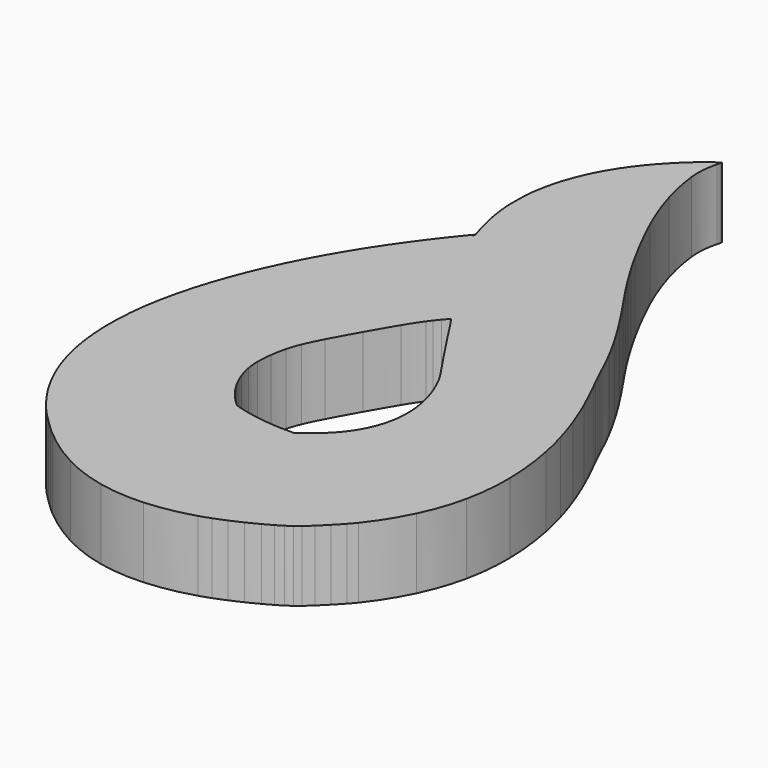
from build123d import *

# Parameters (mm, degrees)
F1_DEPTH = 7


# Not quite as in the source:
# - ends of sketch curves that miss each other by under 0.0002 mm in the source are joined


with BuildPart() as f1:
    # F0 (on Top) → F1 (new body)
    with BuildSketch(Plane.XY):
        with BuildLine():
            ThreePointArc((-0.430785183, 36.1569095573), (-0.5448735218, 36.07329488), (-0.6583357739, 35.9888325768))
            ThreePointArc((-0.6583357739, 35.9888325768), (-0.9799654125, 35.7427966247), (-1.2969257181, 35.4907738493))
            ThreePointArc((-1.2969257181, 35.4907738493), (-1.588219223, 35.2490783173), (-1.8738893459, 35.0007615494))
            ThreePointArc((-1.8738893459, 35.0007615494), (-2.170015105, 34.7316156379), (-2.460329438, 34.4562112538))
            ThreePointArc((-2.460329438, 34.4562112538), (-2.7974429647, 34.1252214563), (-3.1302166301, 33.7898687117))
            ThreePointArc((-3.1302166301, 33.7898687117), (-4.1577341744, 32.6656586922), (-5.1052183742, 31.4732182677))
            ThreePointArc((-5.1052183742, 31.4732182677), (-5.922526202, 30.27128249), (-6.6418773986, 29.0082798961))
            ThreePointArc((-6.6418773986, 29.0082798961), (-7.2424363113, 27.7232778163), (-7.7362109875, 26.3935831428))
            ThreePointArc((-7.7362109875, 26.3935831428), (-8.1209616471, 25.025538406), (-8.3935213198, 23.630801624))
            ThreePointArc((-8.3935213198, 23.630801624), (-8.4452917761, 23.2369178955), (-8.479911135, 22.8411577758))
            ThreePointArc((-8.479911135, 22.8411577758), (-8.5088770783, 22.321651254), (-8.5276155779, 21.8016753695))
            ThreePointArc((-8.5276155779, 21.8016753695), (-8.5362252607, 21.2740019218), (-8.5344179575, 20.7462613338))
            ThreePointArc((-8.5344179575, 20.7462613338), (-8.5208049142, 20.3219677663), (-8.4912689551, 19.8984846225))
            ThreePointArc((-8.4912689551, 19.8984846225), (-8.4359465583, 19.3616858058), (-8.3653124546, 18.8266864033))
            ThreePointArc((-8.3653124546, 18.8266864033), (-8.2793145691, 18.2929917677), (-8.1781847712, 17.7619565862))
            ThreePointArc((-8.1781847712, 17.7619565862), (-8.0586675222, 17.2176479242), (-7.9242287086, 16.6768314139))
            ThreePointArc((-7.9242287086, 16.6768314139), (-7.7675078493, 16.108354433), (-7.5976332474, 15.543668569))
            ThreePointArc((-7.5976332474, 15.543668569), (-7.5308709348, 15.3281742327), (-7.465572902, 15.1122316888))
            ThreePointArc((-7.465572902, 15.1122316888), (-7.4429329744, 15.0246395831), (-7.4268873166, 14.9356031844))
            ThreePointArc((-7.4268873166, 14.9356031844), (-7.4251438345, 14.8835531865), (-7.4345449533, 14.8323295571))
            ThreePointArc((-7.4345449533, 14.8323295571), (-7.4543676211, 14.7885541072), (-7.4852364654, 14.7517255419))
            ThreePointArc((-7.4852364654, 14.7517255419), (-7.5204121413, 14.7198521996), (-7.5556405993, 14.6880372052))
            ThreePointArc((-7.5556405993, 14.6880372052), (-7.5587487588, 14.6866185548), (-7.5621084164, 14.6872397994))
            ThreePointArc((-7.5621084164, 14.6872397994), (-7.5638315071, 14.6895003948), (-7.5632360349, 14.6922797512))
            ThreePointArc((-7.5632360349, 14.6922797512), (-7.5361922486, 14.7283622766), (-7.5090792356, 14.7643928129))
            ThreePointArc((-7.5090792356, 14.7643928129), (-7.4938321529, 14.7858658142), (-7.4798381467, 14.8081757009))
            ThreePointArc((-7.4798381467, 14.8081757009), (-7.4689720046, 14.8285770341), (-7.4598647439, 14.8498219234))
            ThreePointArc((-7.4598647439, 14.8498219234), (-7.4544069217, 14.8666932247), (-7.450657178, 14.8840243528))
            ThreePointArc((-7.450657178, 14.8840243528), (-7.451398276, 14.8940256278), (-7.4566252049, 14.9025844842))
            ThreePointArc((-7.4566252049, 14.9025844842), (-7.4680065339, 14.907037941), (-7.4790015161, 14.9017013868))
            ThreePointArc((-7.4790015161, 14.9017013868), (-7.6134631129, 14.7439014484), (-7.7476745971, 14.5858887302))
            ThreePointArc((-7.7476745971, 14.5858887302), (-7.9002178395, 14.4043837577), (-8.0511495633, 14.2215365248))
            ThreePointArc((-8.0511495633, 14.2215365248), (-8.2291566151, 14.0027594038), (-8.4060060154, 13.7830454333))
            ThreePointArc((-8.4060060154, 13.7830454333), (-10.0845309314, 11.603507652), (-11.6798181849, 9.3623272917))
            ThreePointArc((-11.6798181849, 9.3623272917), (-13.1044368467, 7.1769804809), (-14.4312271442, 4.9308935444))
            ThreePointArc((-14.4312271442, 4.9308935444), (-15.6082959003, 2.716002647), (-16.6822163772, 0.4493029863))
            ThreePointArc((-16.6822163772, 0.4493029863), (-17.6254553738, -1.814282942), (-18.4561232923, -4.1215566279))
            ThreePointArc((-18.4561232923, -4.1215566279), (-19.1707819963, -6.5241501057), (-19.7311264799, -8.9673460764))
            ThreePointArc((-19.7311264799, -8.9673460764), (-20.0884142782, -11.2693053723), (-20.2622984397, -13.5923282872))
            ThreePointArc((-20.2622984397, -13.5923282872), (-20.2459444001, -15.7734645941), (-20.0441447513, -17.9453071175))
            ThreePointArc((-20.0441447513, -17.9453071175), (-19.6631021687, -19.9863200059), (-19.0828292539, -21.9798621794))
            ThreePointArc((-19.0828292539, -21.9798621794), (-18.7353237771, -22.9120276022), (-18.3430469332, -23.8262547684))
            ThreePointArc((-18.3430469332, -23.8262547684), (-17.9051716283, -24.7247504061), (-17.4248569232, -25.6012930339))
            ThreePointArc((-17.4248569232, -25.6012930339), (-16.8987016857, -26.4616549407), (-16.33239559, -27.2961364274))
            ThreePointArc((-16.33239559, -27.2961364274), (-15.7201693746, -28.1137631117), (-15.0713133944, -28.9026358827))
            ThreePointArc((-15.0713133944, -28.9026358827), (-14.8029812176, -29.205115929), (-14.5259723001, -29.4996705008))
            ThreePointArc((-14.5259723001, -29.4996705008), (-14.1382242966, -29.8955327915), (-13.7459105695, -30.2868707615))
            ThreePointArc((-13.7459105695, -30.2868707615), (-13.3369608627, -30.685397769), (-12.9233670761, -31.0791030117))
            ThreePointArc((-12.9233670761, -31.0791030117), (-12.5790868875, -31.3962136045), (-12.2281843577, -31.7059802764))
            ThreePointArc((-12.2281843577, -31.7059802764), (-10.2866629844, -33.2027297), (-8.1902804014, -34.4735342201))
            ThreePointArc((-8.1902804014, -34.4735342201), (-6.1028898704, -35.4062923436), (-3.9072530761, -36.0437999968))
            ThreePointArc((-3.9072530761, -36.0437999968), (-1.665447032, -36.3691333019), (0.5998159048, -36.3800849822))
            ThreePointArc((0.5998159048, -36.3800849822), (2.9747475979, -36.0842879256), (5.298219399, -35.5104628315))
            ThreePointArc((5.298219399, -35.5104628315), (5.8607896787, -35.3267618584), (6.4178395966, -35.1269450508))
            ThreePointArc((6.4178395966, -35.1269450508), (7.0136174484, -34.8957016393), (7.6039516744, -34.6508950513))
            ThreePointArc((7.6039516744, -34.6508950513), (8.2155519266, -34.3810528539), (8.8210819608, -34.0978514095))
            ThreePointArc((8.8210819608, -34.0978514095), (9.4308727796, -33.7965934441), (10.0342530279, -33.482693013))
            ThreePointArc((10.0342530279, -33.482693013), (10.4862467367, -33.237846543), (10.9351066519, -32.9873013725))
            ThreePointArc((10.9351066519, -32.9873013725), (11.2716268321, -32.7902869618), (11.602408112, -32.5837821056))
            ThreePointArc((11.602408112, -32.5837821056), (11.8837105385, -32.3955908709), (12.1583335974, -32.1977799229))
            ThreePointArc((12.1583335974, -32.1977799229), (12.4335473356, -31.9852937195), (12.7018400709, -31.7641331522))
            ThreePointArc((12.7018400709, -31.7641331522), (13.0746340571, -31.436715819), (13.4372173133, -31.0980259196))
            ThreePointArc((13.4372173133, -31.0980259196), (13.8862671378, -30.6588226632), (14.3285485602, -30.2128042907))
            ThreePointArc((14.3285485602, -30.2128042907), (14.7592528316, -29.7649930667), (15.1830855711, -29.3106728376))
            ThreePointArc((15.1830855711, -29.3106728376), (15.4954066752, -28.958764604), (15.7954344436, -28.5963184489))
            ThreePointArc((15.7954344436, -28.5963184489), (17.1719812908, -26.6596111382), (18.3220637149, -24.5804221503))
            ThreePointArc((18.3220637149, -24.5804221503), (19.2039579692, -22.4281271944), (19.8216848423, -20.1856899996))
            ThreePointArc((19.8216848423, -20.1856899996), (20.185400051, -17.8009196363), (20.2734694274, -15.3901807014))
            ThreePointArc((20.2734694274, -15.3901807014), (20.1012942364, -12.7754425625), (19.6955737998, -10.1866415352))
            ThreePointArc((19.6955737998, -10.1866415352), (19.4012368725, -8.8711311402), (19.0550255636, -7.568311292))
            ThreePointArc((19.0550255636, -7.568311292), (18.6471547667, -6.2383521338), (18.1916089548, -4.9239595125))
            ThreePointArc((18.1916089548, -4.9239595125), (17.6536889937, -3.5300826845), (17.0696557218, -2.1548897405))
            ThreePointArc((17.0696557218, -2.1548897405), (16.3778906344, -0.6483852223), (15.6495602976, 0.8407855944))
            ThreePointArc((15.6495602976, 0.8407855944), (15.4915487133, 1.1562432448), (15.3352536377, 1.4725548621))
            ThreePointArc((15.3352536377, 1.4725548621), (15.1623215875, 1.8266905409), (14.9907734063, 2.1814986502))
            ThreePointArc((14.9907734063, 2.1814986502), (14.8288184344, 2.5198460398), (14.6681985189, 2.8588292427))
            ThreePointArc((14.6681985189, 2.8588292427), (14.5461952001, 3.1205105916), (14.4264220559, 3.3832201879))
            ThreePointArc((14.4264220559, 3.3832201879), (13.9049914328, 4.4969156022), (13.3517597861, 5.5951606176))
            ThreePointArc((13.3517597861, 5.5951606176), (12.730347678, 6.7523339658), (12.0817985284, 7.8945192253))
            ThreePointArc((12.0817985284, 7.8945192253), (11.3344304377, 9.1448554979), (10.5608914951, 10.3791720546))
            ThreePointArc((10.5608914951, 10.3791720546), (9.6525095169, 11.7734607934), (8.7244737095, 13.1547458638))
            ThreePointArc((8.7244737095, 13.1547458638), (8.1473512039, 14.0091022489), (7.5780734535, 14.8687056817))
            ThreePointArc((7.5780734535, 14.8687056817), (7.0658883353, 15.6601278636), (6.5632097109, 16.4576219802))
            ThreePointArc((6.5632097109, 16.4576219802), (6.0869127641, 17.2341178808), (5.6203213364, 18.0164842306))
            ThreePointArc((5.6203213364, 18.0164842306), (5.1511799174, 18.8250024409), (4.6913866621, 19.6388731488))
            ThreePointArc((4.6913866621, 19.6388731488), (3.3360934544, 22.1899554001), (2.0846308423, 24.7935455494))
            ThreePointArc((2.0846308423, 24.7935455494), (1.1651287277, 27.0111835931), (0.4023802706, 29.287500229))
            ThreePointArc((0.4023802706, 29.287500229), (-0.0655778033, 31.1552540707), (-0.3715161523, 33.0562777147))
            ThreePointArc((-0.3715161523, 33.0562777147), (-0.4004827326, 34.5139714284), (-0.1486503281, 35.950039133))
            ThreePointArc((-0.1486503281, 35.950039133), (-0.1256281666, 36.0348577325), (-0.10350409, 36.1199150069))
            ThreePointArc((-0.10350409, 36.1199150069), (-0.0855562818, 36.1930052748), (-0.0688372559, 36.2663863711))
            ThreePointArc((-0.0688372559, 36.2663863711), (-0.0553520421, 36.3289076628), (-0.0422658053, 36.3915136791))
            ThreePointArc((-0.0422658053, 36.3915136791), (-0.0427099632, 36.4015567896), (-0.0478641636, 36.4101878819))
            ThreePointArc((-0.0478641636, 36.4101878819), (-0.0563790014, 36.4141917801), (-0.0654906889, 36.411844305))
            ThreePointArc((-0.0654906889, 36.411844305), (-0.1507463247, 36.3535764081), (-0.2358230257, 36.295047559))
            ThreePointArc((-0.2358230257, 36.295047559), (-0.3337291152, 36.2265784006), (-0.430785183, 36.1569095573))
        make_face()
        with BuildLine():
            ThreePointArc((0.7945979778, 1.4604742871), (1.0415519444, 1.0820480924), (1.2874620325, 0.7029427311))
            ThreePointArc((1.2874620779, 0.7029427604), (1.7157577148, 0.043022533), (2.146198459, -0.6155005302))
            ThreePointArc((2.146198433, -0.6155005473), (2.625083452, -1.3436391143), (3.105711714, -2.0706281844))
            ThreePointArc((3.1057117569, -2.0706281559), (3.6027925227, -2.8186455769), (4.101622286, -3.5654977826))
            ThreePointArc((4.1016222508, -3.5654978062), (4.5854050304, -4.2859644865), (5.0710550698, -5.0051738125))
            ThreePointArc((5.0710550942, -5.005173796), (5.2976506486, -5.3552630758), (5.5095035748, -5.7144655073))
            ThreePointArc((5.5095035317, -5.7144655315), (5.7210503835, -6.1063252712), (5.9190958063, -6.505178799))
            ThreePointArc((5.9190958007, -6.5051788017), (6.1121167813, -6.9289171917), (6.2911674393, -7.3587452783))
            ThreePointArc((6.2911674729, -7.358745265), (6.4608873318, -7.8053247091), (6.6169974361, -8.2568417805))
            ThreePointArc((6.6169974071, -8.25684179), (6.943511629, -9.4377235378), (7.1554110445, -10.6444512938))
            ThreePointArc((7.1554110621, -10.6444512916), (7.2291511734, -11.7743743148), (7.1655343607, -12.9049124803))
            ThreePointArc((7.165534362, -12.9049124805), (6.9699742793, -13.9762208263), (6.6399810958, -15.0140309326))
            ThreePointArc((6.6399810845, -15.0140309282), (6.1771168058, -16.0163639167), (5.595527705, -16.9548035143))
            ThreePointArc((5.5955277044, -16.9548035139), (5.3239823263, -17.3157091391), (5.0318840475, -17.660191879))
            ThreePointArc((5.0318840705, -17.6601918998), (4.6740325301, -18.0434743082), (4.3021162058, -18.4131246528))
            ThreePointArc((4.3021162066, -18.4131246536), (3.9089978299, -18.7758402905), (3.5027520416, -19.1237900725))
            ThreePointArc((3.5027520468, -19.1237900787), (3.1215472875, -19.422678131), (2.725970827, -19.7022678306))
            Line((2.7259708143, -19.7022678117), (2.3898394587, -19.9275354802))
            Line((2.3898394587, -19.9275354802), (1.572507513, -19.9275354802))
            ThreePointArc((1.572507513, -19.9275354802), (0.975896833, -19.917051749), (0.3800228029, -19.8856136766))
            ThreePointArc((0.3800228024, -19.8856136843), (-0.2430432422, -19.8321817064), (-0.8641876477, -19.7597531234))
            ThreePointArc((-0.8641876427, -19.7597530856), (-1.4761063823, -19.669303323), (-2.0849488795, -19.5600489544))
            ThreePointArc((-2.0849488781, -19.5600489473), (-2.6483069185, -19.4387928386), (-3.2066394632, -19.2961741329))
            ThreePointArc((-3.2066394768, -19.2961741822), (-3.4512924245, -19.2270775601), (-3.6950806145, -19.1549892361))
            ThreePointArc((-3.6950806131, -19.1549892316), (-3.8079887182, -19.115028714), (-3.9166947744, -19.064748733))
            ThreePointArc((-3.9166947715, -19.0647487274), (-4.0092673629, -19.009250333), (-4.0944900371, -18.9430170162))
            ThreePointArc((-4.0944900381, -18.9430170174), (-4.2290667574, -18.8213648756), (-4.3601783716, -18.6959859236))
            ThreePointArc((-4.3601783887, -18.695985941), (-4.8847775043, -18.1426081191), (-5.3693732956, -17.5538822365))
            ThreePointArc((-5.3693732665, -17.5538822142), (-5.8020023424, -16.9435124036), (-6.1882366718, -16.3027766814))
            ThreePointArc((-6.1882367272, -16.3027767121), (-6.5165955357, -15.652063398), (-6.794495329, -14.9782540563))
            ThreePointArc((-6.7944952456, -14.9782540255), (-7.0109037244, -14.3056858355), (-7.1703984249, -13.6173966227))
            ThreePointArc((-7.1703984556, -13.6173966285), (-7.2608486758, -12.9680544696), (-7.289289434, -12.3130601146))
            ThreePointArc((-7.2892894958, -12.3130601144), (-7.2624894743, -11.5609549338), (-7.1883814889, -10.8120300708))
            ThreePointArc((-7.1883814822, -10.8120300717), (-7.0641246603, -10.0469326426), (-6.892907761, -9.2909573736))
            ThreePointArc((-6.8929077297, -9.2909573817), (-6.6849989692, -8.5981569573), (-6.425145227, -7.9231202815))
            ThreePointArc((-6.425145211, -7.9231202884), (-6.0053130462, -6.999515318), (-5.5466768407, -6.0945523249))
            ThreePointArc((-5.546676867, -6.0945523109), (-4.7895047631, -4.6959164615), (-4.0158876013, -3.3063092072))
            ThreePointArc((-4.0158875933, -3.3063092117), (-3.2252978891, -1.9248741545), (-2.4184162114, -0.5528913355))
            ThreePointArc((-2.4184161815, -0.5528913533), (-1.8764502519, 0.314589724), (-1.2987481474, 1.1586932524))
            ThreePointArc((-1.2987481604, 1.1586932617), (-1.1300178884, 1.3889673688), (-0.9561235489, 1.6153670767))
            ThreePointArc((-0.9561235364, 1.6153670669), (-0.748645804, 1.8753991367), (-0.5374602207, 2.1324289719))
            ThreePointArc((-0.5374602433, 2.1324289907), (-0.3234595466, 2.3881199208), (-0.1084877534, 2.6429949453))
            ThreePointArc((-0.1084877456, 2.6429949387), (-0.0739263748, 2.6693323339), (-0.0314931471, 2.6786901079))
            ThreePointArc((-0.0314931471, 2.6786901079), (-0.0168636226, 2.6750277842), (-0.0056850602, 2.6649047736))
            ThreePointArc((-0.0056850232, 2.6649047984), (0.1837071584, 2.3816563151), (0.372959392, 2.0983143066))
            ThreePointArc((0.3729593742, 2.0983142947), (0.5845013659, 1.7798720187), (0.7945980122, 1.4604743096))
        make_face(mode=Mode.SUBTRACT)
    extrude(amount=F1_DEPTH)


solid = f1.part
